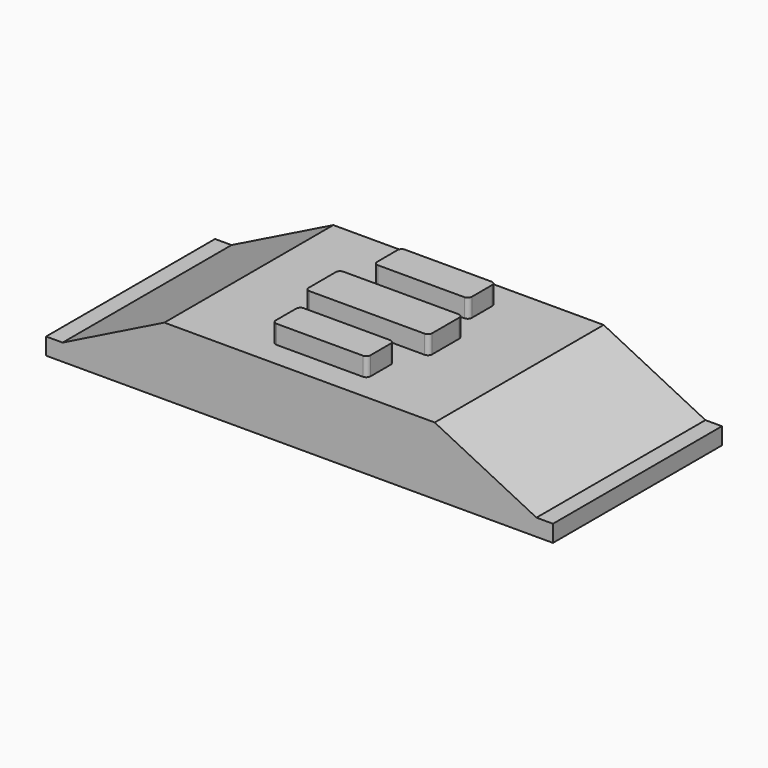
from build123d import *

# Parameters (mm, degrees)
F0_W     = 60
F0_H     = 25
F1_DEPTH = 2
F3_DEPTH = 25
F4_W     = 11.2
F4_H     = 4
F5_DEPTH = 2.2
F6_R     = 0.5


with BuildPart() as f1:
    # F0 (on Top) → F1 (new body)
    with BuildSketch(Plane.XY):
        with Locations((30, 12.5)):
            Rectangle(F0_W, F0_H)
    extrude(amount=F1_DEPTH)

    # F2 (on face) → F3 (join, through all)
    with BuildSketch(Plane(origin=(0, 25, 0), x_dir=(-1, 0, 0), z_dir=(0, 1, 0))):
        Polygon((-1.9529488989, 2), (-14, 8), (-46, 8), (-58.0470511011, 2), align=None)
    extrude(amount=-F3_DEPTH)

    # F4 (on face) → F5 (join)
    with BuildSketch(Plane.XY.offset(8)):
        with Locations((30, 5)):
            Rectangle(F4_W, F4_H)
        Polygon((22.7, 13.0000000004), (22.7, 11.9999999996), (22.7, 10), (37.3, 10), (37.3, 12.5), (37.3, 15), (22.7, 15), align=None)
        with Locations((30, 20)):
            Rectangle(F4_W, F4_H)
    extrude(amount=F5_DEPTH)

    # F6
    f6_edges = [f1.edges().sort_by_distance(p)[0] for p in [
        (24.4, 18, 9.1),
        (35.6, 18, 9.1),
        (22.7, 10, 9.1),
        (24.4, 3, 9.1),
        (35.6, 3, 9.1),
        (22.7, 15, 9.1),
        (35.6, 7, 9.1),
        (24.4, 7, 9.1),
        (24.4, 22, 9.1),
        (35.6, 22, 9.1),
        (37.3, 10, 9.1),
        (37.3, 15, 9.1),
    ]]
    fillet(f6_edges, radius=F6_R)


solid = f1.part
